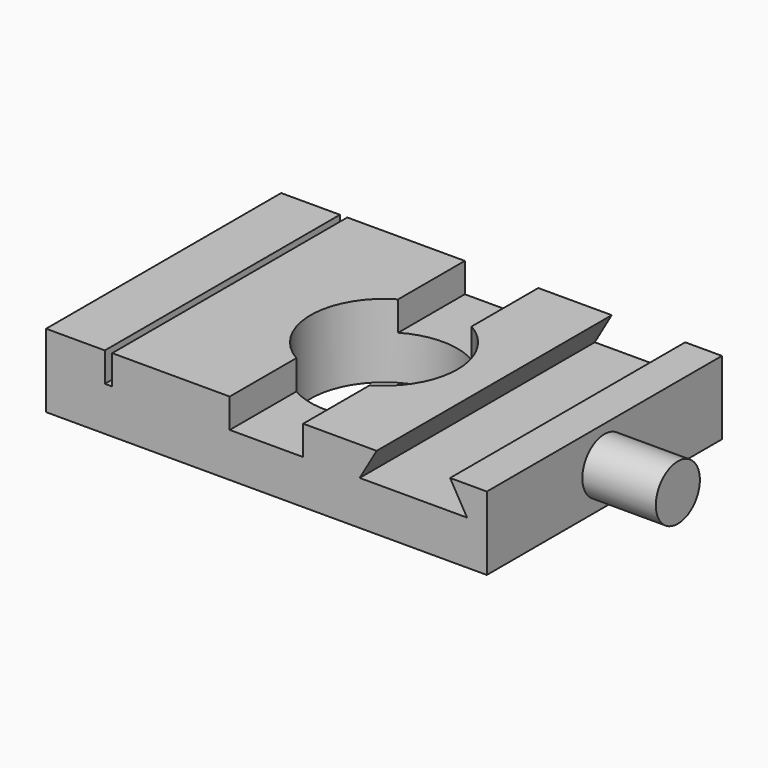
from build123d import *

# Parameters (mm, degrees)
F0_W     = 76.2
F0_H     = 50.8
F0_R     = 12.7
F1_DEPTH = 12.7
F2_W     = 1.27
F2_H     = 50.8
F3_DEPTH = 5.08
F5_DEPTH = 50.801
F6_R     = 4.7625
F7_DEPTH = 12.7


with BuildPart() as f1:
    # F0 (on Top) → F1 (new body)
    with BuildSketch(Plane.XY):
        Rectangle(F0_W, F0_H)
        Circle(F0_R, mode=Mode.SUBTRACT)
    extrude(amount=F1_DEPTH)

    # F2 (on face) → F3 (cut)
    with BuildSketch(Plane.XY.offset(12.7)):
        with Locations((-27.305, 0)):
            Rectangle(F2_W, F2_H)
        with BuildLine():
            Line((-6.35, -10.9985226281), (-6.35, -25.4))
            Line((-6.35, -25.4), (6.35, -25.4))
            Line((6.35, -25.4), (6.35, -10.9985226281))
            ThreePointArc((6.35, -10.9985226281), (0, -12.7), (-6.35, -10.9985226281))
        make_face()
        with BuildLine():
            ThreePointArc((6.35, 10.9985226281), (0, 12.7), (-6.35, 10.9985226281))
            Line((-6.35, 10.9985226281), (-6.35, -10.9985226281))
            ThreePointArc((-6.35, -10.9985226281), (0, -12.7), (6.35, -10.9985226281))
            Line((6.35, -10.9985226281), (6.35, 10.9985226281))
        make_face()
        with BuildLine():
            Line((6.35, 25.4), (-6.35, 25.4))
            Line((-6.35, 25.4), (-6.35, 10.9985226281))
            ThreePointArc((-6.35, 10.9985226281), (0, 12.7), (6.35, 10.9985226281))
            Line((6.35, 10.9985226281), (6.35, 25.4))
        make_face()
    extrude(amount=-F3_DEPTH, mode=Mode.SUBTRACT)

    # F4 (on face) → F5 (cut, through all)
    with BuildSketch(Plane.XZ.offset(25.4)):
        Polygon((31.75, 12.7), (19.05, 12.7), (16.1170606325, 7.62), (34.6829393675, 7.62), align=None)
    extrude(amount=-F5_DEPTH, mode=Mode.SUBTRACT)

    # F6 (on face) → F7 (join)
    with BuildSketch(Plane.YZ.offset(38.1)):
        with Locations((0, 6.35)):
            Circle(F6_R)
    extrude(amount=F7_DEPTH)


solid = f1.part
